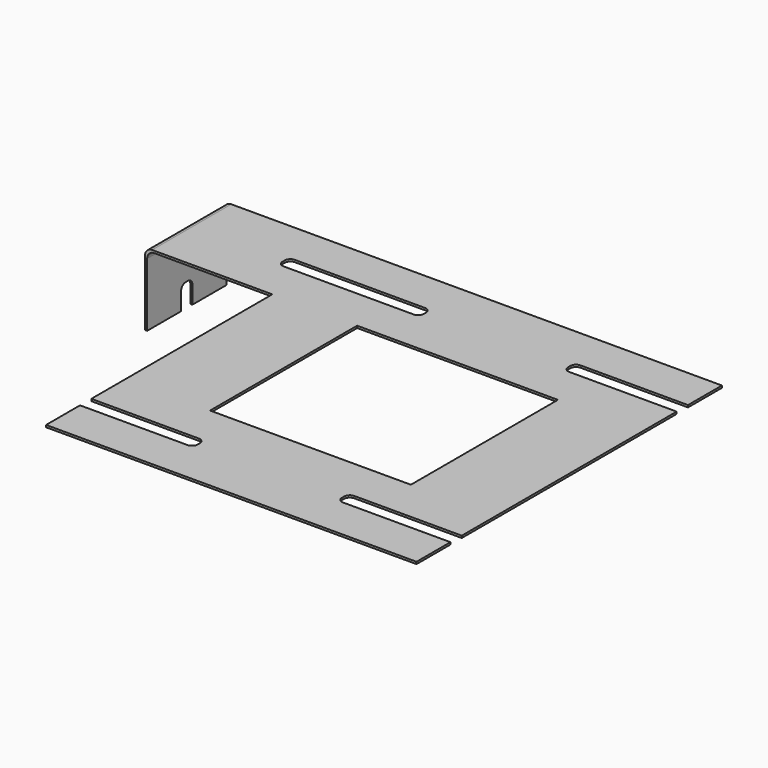
from build123d import *

# Parameters (mm, degrees)
F0_W     = 14.2
F0_H     = 13
F1_DEPTH = 0.15
F2_W     = 0.15
F2_H     = 7
F3_DEPTH = 5
F4_R     = 0.5
F6_DEPTH = 25


# Not quite as in the source:
# - a feature names something its author has since deleted; it is built from what else it names


with BuildPart() as f1:
    # F0 (on Top) → F1 (new body)
    with BuildSketch(Plane.XY):
        with BuildLine():
            Line((-13.1, 10.5), (-13.1, 13.5))
            Line((-13.1, 13.5), (-22.1, 13.5))
            Line((-22.1, 13.5), (-22.1, 6.5))
            Line((-22.1, 6.5), (-13.1, 6.5))
            Line((-13.1, 6.5), (-13.1, 9.5))
            Line((-13.1, 9.5), (-14.7, 9.5))
            ThreePointArc((-14.7, 9.5), (-14.9828427125, 9.6171572875), (-15.1, 9.9))
            Line((-15.1, 9.9), (-15.1, 10.1))
            ThreePointArc((-15.1, 10.1), (-14.9828427125, 10.3828427125), (-14.7, 10.5))
            Line((-14.7, 10.5), (-13.1, 10.5))
        make_face()
        with BuildLine():
            Line((13.1, 10.5), (13.1, 13.5))
            Line((13.1, 13.5), (-7.1, 13.5))
            Line((-7.1, 13.5), (-13.1, 13.5))
            Line((-13.1, 13.5), (-13.1, 10.5))
            Line((-13.1, 10.5), (-5.5, 10.5))
            ThreePointArc((-5.5, 10.5), (-5.2171572875, 10.3828427125), (-5.1, 10.1))
            Line((-5.1, 10.1), (-5.1, 9.9))
            ThreePointArc((-5.1, 9.9), (-5.2171572875, 9.6171572875), (-5.5, 9.5))
            Line((-5.5, 9.5), (-13.1, 9.5))
            Line((-13.1, 9.5), (-13.1, 6.5))
            Line((-13.1, 6.5), (-13.1, 0))
            Line((-13.1, 0), (-13.1, -6.5))
            Line((-13.1, -6.5), (-13.1, -9.5))
            Line((-13.1, -9.5), (-5.5, -9.5))
            ThreePointArc((-5.5, -9.5), (-5.2171572875, -9.6171572875), (-5.1, -9.9))
            Line((-5.1, -9.9), (-5.1, -10.1))
            ThreePointArc((-5.1, -10.1), (-5.2171572875, -10.3828427125), (-5.5, -10.5))
            Line((-5.5, -10.5), (-13.1, -10.5))
            Line((-13.1, -10.5), (-13.1, -13.5))
            Line((-13.1, -13.5), (-7.1, -13.5))
            Line((-7.1, -13.5), (13.1, -13.5))
            Line((13.1, -13.5), (13.1, -10.5))
            Line((13.1, -10.5), (5.5, -10.5))
            ThreePointArc((5.5, -10.5), (5.2171572875, -10.3828427125), (5.1, -10.1))
            Line((5.1, -10.1), (5.1, -9.9))
            ThreePointArc((5.1, -9.9), (5.2171572875, -9.6171572875), (5.5, -9.5))
            Line((5.5, -9.5), (13.1, -9.5))
            Line((13.1, -9.5), (13.1, 0))
            Line((13.1, 0), (13.1, 9.5))
            Line((13.1, 9.5), (5.5, 9.5))
            ThreePointArc((5.5, 9.5), (5.2171572875, 9.6171572875), (5.1, 9.9))
            Line((5.1, 9.9), (5.1, 10.1))
            ThreePointArc((5.1, 10.1), (5.2171572875, 10.3828427125), (5.5, 10.5))
            Line((5.5, 10.5), (13.1, 10.5))
        make_face()
        Rectangle(F0_W, F0_H, mode=Mode.SUBTRACT)
    extrude(amount=F1_DEPTH)

    # F2 (on face) → F3 (join)
    with BuildSketch(Plane(origin=(0, 0, 0), x_dir=(1, 0, 0), z_dir=(0, 0, -1))):
        with Locations((-22.025, -10)):
            Rectangle(F2_W, F2_H)
    extrude(amount=F3_DEPTH)

    # F4
    f4_edges = [f1.edges().sort_by_distance(p)[0] for p in [
        (-21.95, 10, 0),
        (-22.1, 10, 0.15),
    ]]
    fillet(f4_edges, radius=F4_R)

    # F5 (on face) → F6 (cut)
    with BuildSketch(Plane(origin=(-22.1, 0, 0), x_dir=(0, -1, 0), z_dir=(-1, 0, 0))):
        with BuildLine():
            Line((-9.9, -3.35), (-10, -3.35))
            Line((-10, -3.35), (-10.1, -3.35))
            ThreePointArc((-10.1, -3.35), (-10.3828427125, -3.4671572875), (-10.5, -3.75))
            Line((-10.5, -3.75), (-10.5, -5))
            Line((-10.5, -5), (-9.5, -5))
            Line((-9.5, -5), (-9.5, -3.75))
            ThreePointArc((-9.5, -3.75), (-9.6171572875, -3.4671572875), (-9.9, -3.35))
        make_face()
    extrude(amount=-F6_DEPTH, mode=Mode.SUBTRACT)


solid = f1.part
